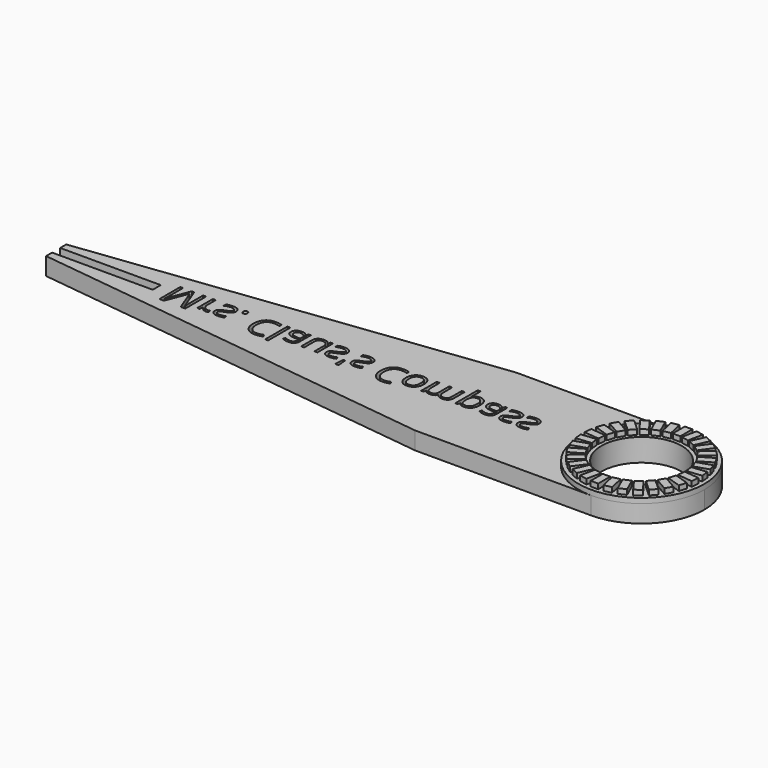
from build123d import *

# Parameters (mm, degrees)
F0_R         = 8
F1_DEPTH     = 3.5
F4_W         = 20
F4_H         = 2
F5_DEPTH     = 2
F2_R         = 12.5
F2_R_2       = 8
F6_DEPTH     = 1
F7_W         = 1.5
F7_H         = 3
F8_DEPTH     = 1
F9_TEXT_SIZE = 7.2601012006
F10_DEPTH    = 5.501


# Not quite as in the source:
# - a feature names something its author has since deleted; it is built from what else it names
# - Text() gives the source's letters only with a copy of the font that has no kerning and outlines rounded to 1/6400 em; it was checked with that copy


with BuildPart() as f1:
    # F0 (on Top) → F1 (new body)
    with BuildSketch(Plane.XY):
        with BuildLine():
            ThreePointArc((0, -12.5), (8.8388347648, -8.8388347648), (12.5, 0))
            ThreePointArc((12.5, 0), (8.8388347648, 8.8388347648), (0, 12.5))
            ThreePointArc((0, 12.5), (-12.5, 0), (0, -12.5))
        make_face()
        Circle(F0_R, mode=Mode.SUBTRACT)
        with BuildLine():
            ThreePointArc((0, -12.5), (-12.5, 0), (0, 12.5))
            Line((0, 12.5), (-35, 12.5))
            Line((-35, 12.5), (-116.3887844346, 2.5067138408))
            Line((-116.3887844346, 2.5067138408), (-116.3887844346, -2.5067138408))
            Line((-116.3887844346, -2.5067138408), (-35, -12.5))
            Line((-35, -12.5), (0, -12.5))
        make_face()
    extrude(amount=F1_DEPTH)

    # F4 (on face) → F5 (cut)
    with BuildSketch(Plane.XY.offset(3.5)):
        with Locations((-106.3887844346, -0.0067138408)):
            Rectangle(F4_W, F4_H)
    extrude(amount=-F5_DEPTH, mode=Mode.SUBTRACT)

    # F2 (on face) → F6 (join)
    with BuildSketch(Plane.XY.offset(3.5)):
        Circle(F2_R)
        Circle(F2_R_2, mode=Mode.SUBTRACT)
    extrude(amount=F6_DEPTH)

    # F7 (on face) → F8 (join)
    with BuildSketch(Plane.XY.offset(4.5)):
        with Locations((0.0070165292, 10.1940347813)):
            Rectangle(F7_W, F7_H)
        Polygon((-1.6908526421, 11.5958846508), (-3.1580740432, 11.2840171146), (-2.5343389708, 8.3495743124), (-1.0671175697, 8.6614418486), align=None)
        Polygon((-4.0648234394, 10.9909387178), (-5.4351416258, 10.3808337532), (-4.2149316966, 7.6401973803), (-2.8446135102, 8.2503023449), align=None)
        Polygon((-6.2611419471, 9.9056360225), (-7.4746674387, 9.023958144), (-5.7113116818, 6.5969071609), (-4.4977861903, 7.4785850394), align=None)
        Polygon((-8.1838185075, 8.3874095004), (-9.187514417, 7.2726922622), (-6.9580799406, 5.2653004432), (-5.9543840311, 6.3800176814), align=None)
        Polygon((-9.7488229288, 6.502612936), (-10.4988229288, 5.2035748303), (-7.9007467174, 3.7035748303), (-7.1507467174, 5.002612936), align=None)
        Polygon((-10.887757008, 4.3336209832), (-11.3512824996, 2.9070362088), (-8.4981129507, 1.9799852257), (-8.0345874591, 3.4065700001), align=None)
        Polygon((-11.5508438607, 1.9752289985), (-11.7076365556, 0.4834461554), (-8.7240708695, 0.1698607656), (-8.5672781746, 1.6616436087), align=None)
        Polygon((-11.7091034097, -0.4694899717), (-11.5523107148, -1.9612728147), (-8.5687450287, -1.6476874249), (-8.7255377236, -0.1559045819), align=None)
        Polygon((-11.3556189531, -2.8936899772), (-10.8920934615, -4.3202747517), (-8.0389239126, -3.3932237685), (-8.5024494042, -1.9666389941), align=None)
        Polygon((-10.5058394579, -5.1914218453), (-9.7558394579, -6.490459951), (-7.1577632466, -4.990459951), (-7.9077632466, -3.6914218453), align=None)
        Polygon((-9.1969043659, -7.2622636675), (-8.1932084563, -8.3769809058), (-5.9637739799, -6.3695890867), (-6.9674698894, -5.2548718485), align=None)
        Polygon((-7.4860204214, -9.0157097193), (-6.2724949298, -9.8973875977), (-4.5091391729, -7.4703366146), (-5.7226646645, -6.5886587362), align=None)
        Polygon((-5.4479614625, -10.3751259942), (-4.0776432761, -10.9852309588), (-2.8574333469, -8.2445945858), (-4.2277515333, -7.6344896212), align=None)
        Polygon((-3.1718004456, -11.2810994777), (-1.7045790445, -11.5929670139), (-1.080843972, -8.6585242117), (-2.5480653731, -8.3466566755), align=None)
        with Locations((-0.0070165292, -10.1940347813)):
            Rectangle(F7_W, F7_H)
        Polygon((1.6908526421, -11.5958846508), (3.1580740432, -11.2840171146), (2.5343389708, -8.3495743124), (1.0671175697, -8.6614418486), align=None)
        Polygon((4.0648234394, -10.9909387178), (5.4351416258, -10.3808337532), (4.2149316966, -7.6401973803), (2.8446135102, -8.2503023449), align=None)
        Polygon((6.2611419471, -9.9056360225), (7.4746674387, -9.023958144), (5.7113116818, -6.5969071609), (4.4977861903, -7.4785850394), align=None)
        Polygon((8.1838185075, -8.3874095004), (9.187514417, -7.2726922622), (6.9580799406, -5.2653004432), (5.9543840311, -6.3800176814), align=None)
        Polygon((9.7488229288, -6.502612936), (10.4988229288, -5.2035748303), (7.9007467174, -3.7035748303), (7.1507467174, -5.002612936), align=None)
        Polygon((10.887757008, -4.3336209832), (11.3512824996, -2.9070362088), (8.4981129507, -1.9799852257), (8.0345874591, -3.4065700001), align=None)
        Polygon((11.5508438607, -1.9752289985), (11.7076365556, -0.4834461554), (8.7240708695, -0.1698607656), (8.5672781746, -1.6616436087), align=None)
        Polygon((11.7091034097, 0.4694899717), (11.5523107148, 1.9612728147), (8.5687450287, 1.6476874249), (8.7255377236, 0.1559045819), align=None)
        Polygon((11.3556189531, 2.8936899772), (10.8920934615, 4.3202747517), (8.0389239126, 3.3932237685), (8.5024494042, 1.9666389941), align=None)
        Polygon((10.5058394579, 5.1914218453), (9.7558394579, 6.490459951), (7.1577632466, 4.990459951), (7.9077632466, 3.6914218453), align=None)
        Polygon((9.1969043659, 7.2622636675), (8.1932084563, 8.3769809058), (5.9637739799, 6.3695890867), (6.9674698894, 5.2548718485), align=None)
        Polygon((7.4860204214, 9.0157097193), (6.2724949298, 9.8973875977), (4.5091391729, 7.4703366146), (5.7226646645, 6.5886587362), align=None)
        Polygon((5.4479614625, 10.3751259942), (4.0776432761, 10.9852309588), (2.8574333469, 8.2445945858), (4.2277515333, 7.6344896212), align=None)
        Polygon((3.1718004456, 11.2810994777), (1.7045790445, 11.5929670139), (1.080843972, 8.6585242117), (2.5480653731, 8.3466566755), align=None)
    extrude(amount=F8_DEPTH)

    # F9 (on face) → F10 (cut, through all)
    with BuildSketch(Plane(origin=(0, 0, 0), x_dir=(1, 0, 0), z_dir=(0, 0, -1))):
        with Locations((-94.3307578564, -2.3863636889)):
            Text("Mrs. Claus's Compass", F9_TEXT_SIZE, font='Open Sans', text_align=(TextAlign.LEFT, TextAlign.BOTTOM))
    extrude(amount=-F10_DEPTH, mode=Mode.SUBTRACT)


solid = f1.part
